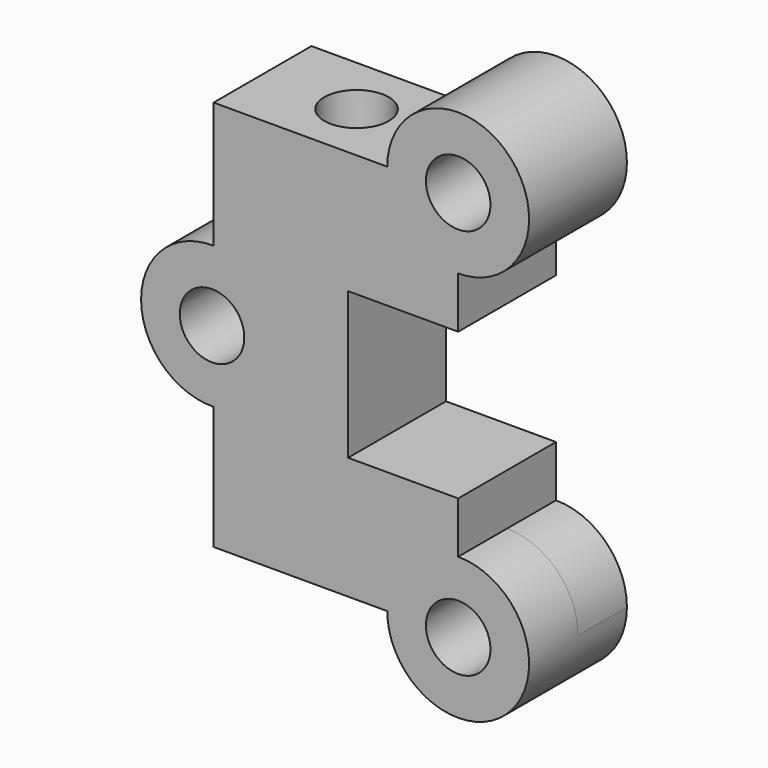
from build123d import *

# Parameters (mm, degrees)
F1_DEPTH       = 12.5
F3_D           = 13.2
F3_CBORE_D     = 19.25
F3_CBORE_DEPTH = 0
F5_D           = 13.2
F5_CBORE_D     = 19.25
F5_CBORE_DEPTH = 0
F6_W           = 45
F6_H           = 30
F7_DEPTH       = 30


with BuildPart() as f1:
    # F0 (on Front) → F1 (new body, symmetric)
    with BuildSketch(Plane.XZ):
        with BuildLine():
            Line((25, -25.5), (25, -40))
            Line((25, -40), (10.5, -40))
            ThreePointArc((10.5, -40), (25, -54.5), (39.5, -40))
            ThreePointArc((39.5, -40), (35.2530483272, -29.7469516728), (25, -25.5))
        make_face()
        with BuildLine():
            Line((10.5, -40), (25, -40))
            Line((25, -40), (25, -25.5))
            ThreePointArc((25, -25.5), (14.7469516728, -29.7469516728), (10.5, -40))
        make_face()
        with BuildLine():
            Line((-25, -40), (10.5, -40))
            ThreePointArc((10.5, -40), (14.7469516728, -29.7469516728), (25, -25.5))
            Line((25, -25.5), (25, 25.5))
            ThreePointArc((25, 25.5), (14.7469516728, 29.7469516728), (10.5, 40))
            Line((10.5, 40), (-25, 40))
            Line((-25, 40), (-25, 14.2162181315))
            ThreePointArc((-25, 14.2162181315), (-14.9640357801, 9.8540823977), (-10.8347666082, -0.279916916))
            ThreePointArc((-10.8347666082, -0.279916916), (-14.9640357801, -10.4139162298), (-25, -14.7760519636))
            Line((-25, -14.7760519636), (-25, -40))
        make_face()
        with BuildLine():
            ThreePointArc((10.5, 40), (14.7469516728, 29.7469516728), (25, 25.5))
            Line((25, 25.5), (25, 40))
            Line((25, 40), (10.5, 40))
        make_face()
        with BuildLine():
            Line((25, 40), (25, 25.5))
            ThreePointArc((25, 25.5), (35.2530483272, 29.7469516728), (39.5, 40))
            ThreePointArc((39.5, 40), (25, 54.5), (10.5, 40))
            Line((10.5, 40), (25, 40))
        make_face()
        with BuildLine():
            ThreePointArc((-25, 14.2162181315), (-39.8347666082, -0.279916916), (-25, -14.7760519636))
            Line((-25, -14.7760519636), (-25, 14.2162181315))
        make_face()
        with BuildLine():
            Line((-25, 14.2162181315), (-25, -14.7760519636))
            ThreePointArc((-25, -14.7760519636), (-14.9640357801, -10.4139162298), (-10.8347666082, -0.279916916))
            ThreePointArc((-10.8347666082, -0.279916916), (-14.9640357801, 9.8540823977), (-25, 14.2162181315))
        make_face()
    extrude(amount=F1_DEPTH, both=True)

    # F3 (through all)
    with Locations(Plane.XZ.offset(12.5)):
        with Locations((25, 40), (-25.3347666082, -0.279916916), (25, -40)):
            CounterBoreHole(F3_D / 2, F3_CBORE_D / 2, F3_CBORE_DEPTH)

    # F5 (through all)
    with Locations(Plane.XY.offset(40)):
        with Locations((-5.7768835686, 0)):
            CounterBoreHole(F5_D / 2, F5_CBORE_D / 2, F5_CBORE_DEPTH)

    # F6 (on face) → F7 (cut)
    with BuildSketch(Plane.XZ.offset(12.5)):
        with Locations((25, 0)):
            Rectangle(F6_W, F6_H)
    extrude(amount=-F7_DEPTH, mode=Mode.SUBTRACT)


solid = f1.part
